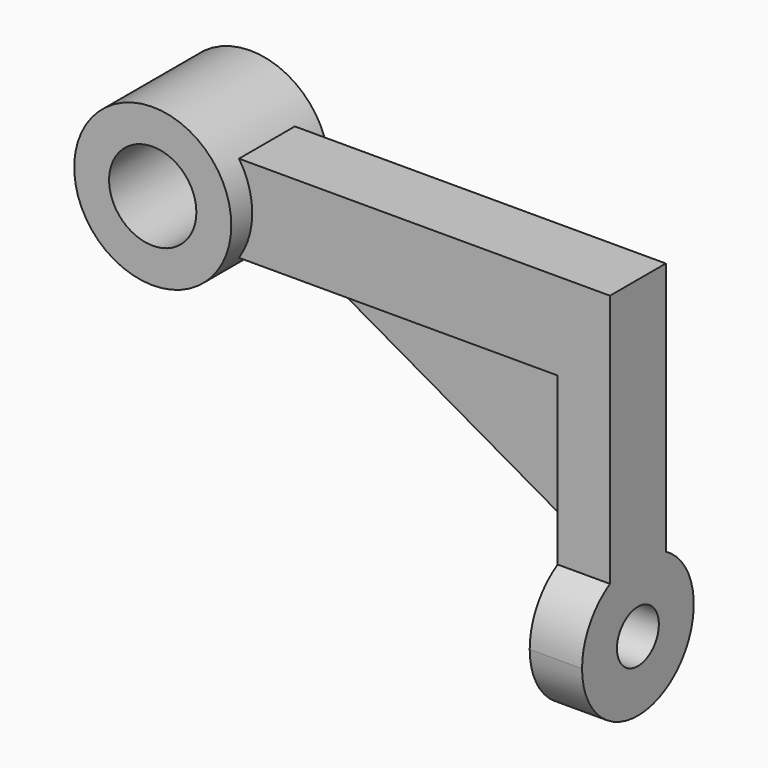
from build123d import *

# Parameters (mm, degrees)
F0_R     = 2.5
F1_DEPTH = 3.5
F2_DEPTH = 2
F4_DEPTH = 3
F6_D     = 3
F8_DEPTH = 1


with BuildPart() as f1:
    # F0 (on Front) → F1 (new body, symmetric)
    with BuildSketch(Plane.XZ):
        with BuildLine():
            Line((-15.9480972197, 5), (-16.6897546064, 5))
            Line((-16.6897546064, 5), (-16.6897546064, 0))
            Line((-16.6897546064, 0), (-15.9480972197, 0))
            ThreePointArc((-15.9480972197, 0), (-15.3835115664, 1.1937569599), (-15.1897546064, 2.5))
            ThreePointArc((-15.1897546064, 2.5), (-15.3835115664, 3.8062430401), (-15.9480972197, 5))
        make_face()
        with BuildLine():
            Line((-16.6897546064, 0), (-16.6897546064, 5))
            Line((-16.6897546064, 5), (-15.9480972197, 5))
            ThreePointArc((-15.9480972197, 5), (-24.1897546064, 2.5), (-15.9480972197, 0))
            Line((-15.9480972197, 0), (-16.6897546064, 0))
        make_face()
        with Locations((-19.6897546064, 2.5)):
            Circle(F0_R, mode=Mode.SUBTRACT)
    extrude(amount=F1_DEPTH, both=True)

    # F0 (on Front) → F2 (join, symmetric)
    with BuildSketch(Plane.XZ):
        with BuildLine():
            Line((-16.6897546064, 0), (-16.6897546064, 5))
            Line((-16.6897546064, 5), (-15.9480972197, 5))
            ThreePointArc((-15.9480972197, 5), (-24.1897546064, 2.5), (-15.9480972197, 0))
            Line((-15.9480972197, 0), (-16.6897546064, 0))
        make_face()
        with Locations((-19.6897546064, 2.5)):
            Circle(F0_R, mode=Mode.SUBTRACT)
        with BuildLine():
            Line((-15.9480972197, 5), (-16.6897546064, 5))
            Line((-16.6897546064, 5), (-16.6897546064, 0))
            Line((-16.6897546064, 0), (-15.9480972197, 0))
            ThreePointArc((-15.9480972197, 0), (-15.3835115664, 1.1937569599), (-15.1897546064, 2.5))
            ThreePointArc((-15.1897546064, 2.5), (-15.3835115664, 3.8062430401), (-15.9480972197, 5))
        make_face()
        with BuildLine():
            Line((5.3102453936, 5), (-15.9480972197, 5))
            ThreePointArc((-15.9480972197, 5), (-15.3835115664, 3.8062430401), (-15.1897546064, 2.5))
            ThreePointArc((-15.1897546064, 2.5), (-15.3835115664, 1.1937569599), (-15.9480972197, 0))
            Line((-15.9480972197, 0), (2.3102453936, 0))
            Line((2.3102453936, 0), (2.3102453936, -15))
            Line((2.3102453936, -15), (5.3102453936, -15))
            Line((5.3102453936, -15), (5.3102453936, 5))
        make_face()
    extrude(amount=F2_DEPTH, both=True)

    # F3 (on face) → F4 (join)
    with BuildSketch(Plane(origin=(2.3102453936, 0, 0), x_dir=(0, -1, 0), z_dir=(-1, 0, 0))):
        with BuildLine():
            ThreePointArc((-2, -9.5358983849), (-2, -16.4641016151), (4, -13))
            ThreePointArc((4, -13), (3.4641016151, -11), (2, -9.5358983849))
            Line((2, -9.5358983849), (2, -15))
            Line((2, -15), (-2, -15))
            Line((-2, -15), (-2, -9.5358983849))
        make_face()
        with BuildLine():
            Line((2, -15), (2, -9.5358983849))
            ThreePointArc((2, -9.5358983849), (0, -9), (-2, -9.5358983849))
            Line((-2, -9.5358983849), (-2, -15))
            Line((-2, -15), (2, -15))
        make_face()
    extrude(amount=-F4_DEPTH)

    # F6 (through all)
    with Locations(Plane(origin=(2.3102453936, 0, 0), x_dir=(0, -1, 0), z_dir=(-1, 0, 0))):
        with Locations((0, -13)):
            Hole(F6_D / 2)

    # F7 (on Front) → F8 (join, symmetric)
    with BuildSketch(Plane.XZ):
        Polygon((2.3102453936, 0), (-11.6897546064, 0), (2.3102453936, -8), align=None)
    extrude(amount=F8_DEPTH, both=True)


solid = f1.part
